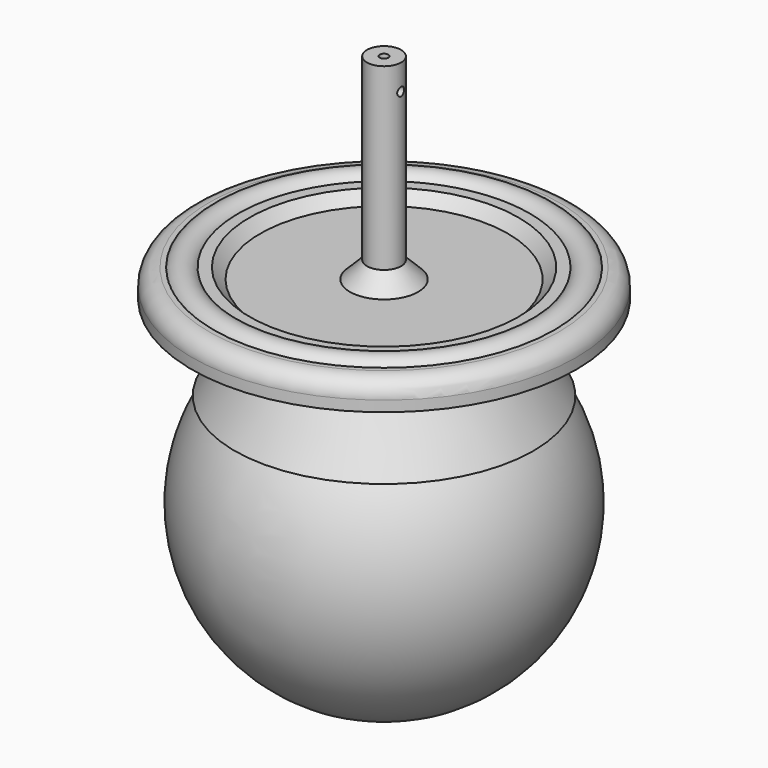
from build123d import *

# Parameters (mm, degrees)
F0_R      = 22.5
F0_R_2    = 16.5
F0_R_3    = 2
F0_R_4    = 0.5
F1_DEPTH  = 2
F2_DEPTH  = 25
F3_DEPTH  = 3.25
F6_R      = 1.75
F10_R     = 2
F11_R     = 17.5
F11_R_2   = 0.5
F12_DEPTH = 10
F15_SIZE2 = 5.773493
F15_SIZE  = 9.99999
F17_R     = 0.5
F18_DEPTH = 12.5


# Not quite as in the source:
# - a fillet or chamfer that OpenCascade refuses, or shapes differently, is made with other operations: its cross-section is extruded or revolved along the edge and cut away or added
# - a fillet or chamfer is up to 0.001 mm smaller than in the source, because OpenCascade refuses the exact size


with BuildPart() as f1:
    # F0 (on Top) → F1 (new body)
    with BuildSketch(Plane.XY):
        Circle(F0_R)
        Circle(F0_R_2, mode=Mode.SUBTRACT)
        Circle(F0_R_2)
        Circle(F0_R_3, mode=Mode.SUBTRACT)
        Circle(F0_R_3)
        Circle(F0_R_4, mode=Mode.SUBTRACT)
    extrude(amount=F1_DEPTH)

    # F0 (on Top) → F2 (join)
    with BuildSketch(Plane.XY):
        Circle(F0_R_3)
        Circle(F0_R_4, mode=Mode.SUBTRACT)
    extrude(amount=F2_DEPTH)

    # F0 (on Top) → F3 (join)
    with BuildSketch(Plane.XY):
        Circle(F0_R)
        Circle(F0_R_2, mode=Mode.SUBTRACT)
    extrude(amount=F3_DEPTH)


with BuildPart() as f7:
    # F6 (on Right) → F7 (revolve)
    with BuildSketch(Plane.YZ):
        with Locations((-18.5, 2.25)):
            Circle(F6_R)
    revolve(axis=Axis((0, 0, 2.25), (0, 0, -1)))


with BuildPart() as f1_1:
    add(f1.part)

    # F8: cut F7
    add(f7.part, mode=Mode.SUBTRACT)

    # F9: chamfer of 2 on 2 edges, made by hand

    # F9_s1 → F9_t2 (revolve)
    with BuildSketch(Plane.XZ):
        Polygon((2, 4), (4, 2), (2, 2), align=None)
    revolve(axis=Axis((0, 0, 2), (0, 0, -1)))


with BuildPart() as f9_tool4:
    # F9_s5 → F9_t6 (revolve)
    with BuildSketch(Plane.XZ):
        Polygon((14.5, 2), (16.5, 4), (16.5, 2), align=None)
    revolve(axis=Axis((0, 0, 2), (0, 0, -1)))

    split(bisect_by=Plane.XY.offset(3.25), keep=Keep.BOTTOM)


with BuildPart() as f1_2:
    add(f1_1.part)

    # F9_t3: union F9_tool4
    add(f9_tool4.part)

    # F10
    f10_edges = [f1_2.edges().sort_by_distance(p)[0] for p in [
        (-22.5, 0, 3.25),
    ]]
    fillet(f10_edges, radius=F10_R)

    # F17 (on Right) → F18 (cut, symmetric)
    with BuildSketch(Plane.YZ):
        with Locations((0, 22)):
            Circle(F17_R)
    extrude(amount=F18_DEPTH, both=True, mode=Mode.SUBTRACT)


with BuildPart() as f12:
    # F11 (on face) → F12 (new body)
    with BuildSketch(Plane(origin=(0, 0, 0), x_dir=(1, 0, 0), z_dir=(0, 0, -1))):
        Circle(F11_R)
        Circle(F11_R_2, mode=Mode.SUBTRACT)
    extrude(amount=F12_DEPTH)

    # F15 (size 10 and 5.7735026919 in the source; OpenCascade refuses exactly that, so slightly less here)
    f15_edges = [f12.edges().sort_by_distance(p)[0] for p in [
        (-17.5, 0, 0),
    ]]
    f15_side = f12.faces().sort_by_distance((-17.5, 0, -5))[0]
    chamfer(f15_edges, length=F15_SIZE, length2=F15_SIZE2, reference=f15_side)


with BuildPart() as f14:
    # F13 (on Right) → F14 (revolve)
    with BuildSketch(Plane.YZ):
        with BuildLine():
            ThreePointArc((0, -0.9), (-20.1, -21), (0, -41.1))
            Line((0, -41.1), (0, -21))
            Line((0, -21), (0, -0.9))
        make_face()
    revolve(axis=Axis((0, 0, -10.5), (0, 0, 1)))


with BuildPart() as f12_1:
    add(f12.part)

    # F16: cut F14
    add(f14.part, mode=Mode.SUBTRACT)


solid = Compound([f7.part, f1_2.part, f14.part, f12_1.part])
